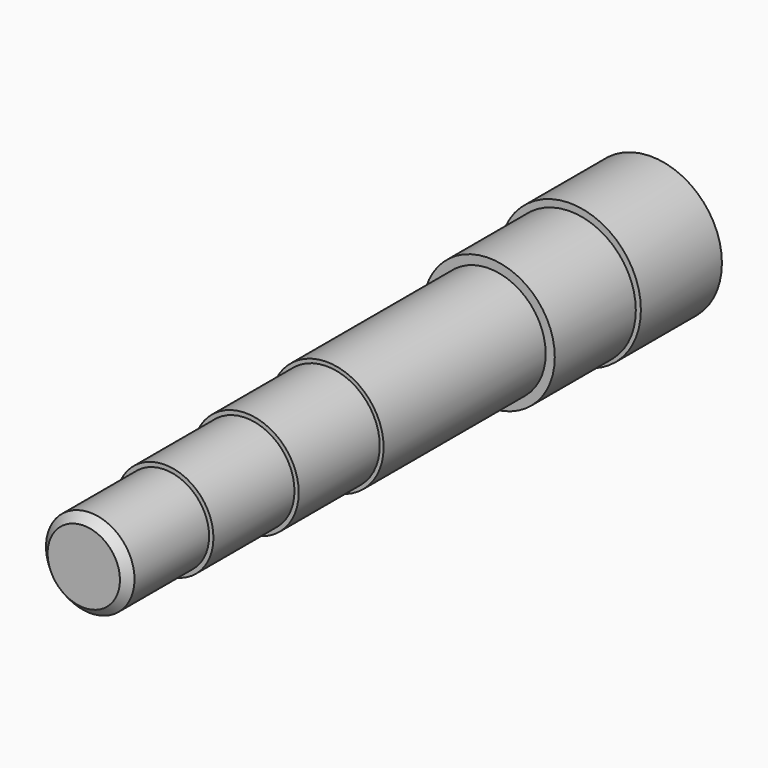
from build123d import *

# Parameters (mm, degrees)
F0_R      = 17.5
F1_DEPTH  = 25
F2_R      = 16.25
F3_DEPTH  = 50
F4_R      = 14
F5_DEPTH  = 100
F6_R      = 13.05
F7_DEPTH  = 125
F8_R      = 12
F9_DEPTH  = 150
F10_R     = 10.925
F11_DEPTH = 175
F12_SIZE  = 2


with BuildPart() as f1:
    # F0 (on Front) → F1 (new body)
    with BuildSketch(Plane.XZ):
        with Locations((0, 0.5113246338)):
            Circle(F0_R)
    extrude(amount=F1_DEPTH)

    # F4 (on Front) → F5 (join)
    with BuildSketch(Plane.XZ):
        Circle(F4_R)
    extrude(amount=F5_DEPTH)

    # F6 (on Front) → F7 (join)
    with BuildSketch(Plane.XZ):
        Circle(F6_R)
    extrude(amount=F7_DEPTH)

    # F8 (on Front) → F9 (join)
    with BuildSketch(Plane.XZ):
        Circle(F8_R)
    extrude(amount=F9_DEPTH)


with BuildPart() as f3:
    # F2 (on Front) → F3 (new body)
    with BuildSketch(Plane.XZ):
        Circle(F2_R)
    extrude(amount=F3_DEPTH)


with BuildPart() as f11:
    # F10 (on Front) → F11 (new body)
    with BuildSketch(Plane.XZ):
        Circle(F10_R)
    extrude(amount=F11_DEPTH)

    # F12
    f12_edges = [f11.edges().sort_by_distance(p)[0] for p in [
        (-10.925, -175, 0),
    ]]
    chamfer(f12_edges, length=F12_SIZE)


solid = Compound([f1.part, f3.part, f11.part])
